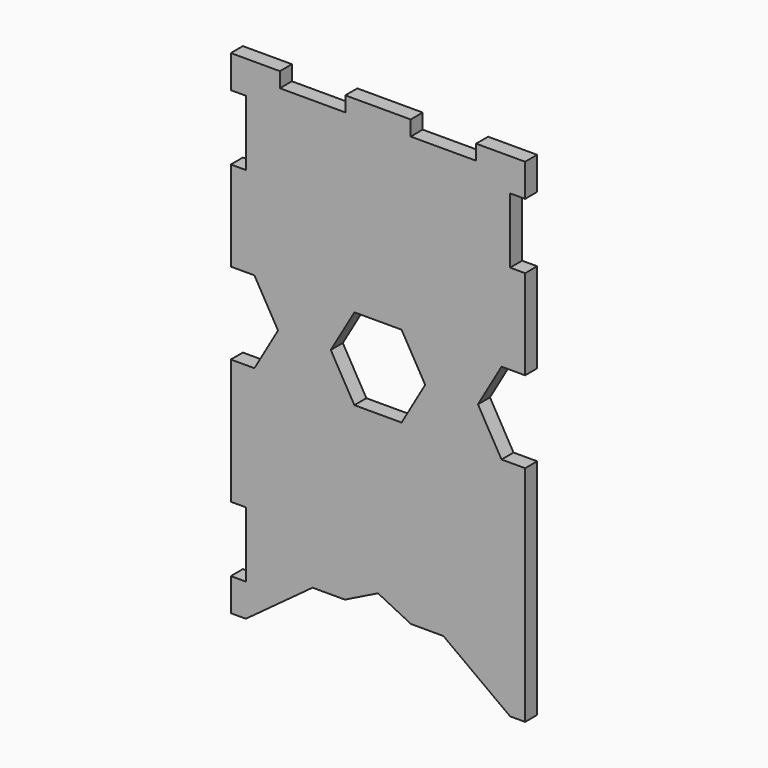
from build123d import *

# Parameters (mm, degrees)
F0_W     = 114.3
F0_H     = 191.516
F1_DEPTH = 5.842
F2_W     = 5.842
F2_H     = 25.4
F2_W_2   = 25.4
F2_H_2   = 5.842
F3_DEPTH = 5.842
F5_DEPTH = 5.842


# Not quite as in the source:
# - a feature names something its author has since deleted; it is built from what else it names


with BuildPart() as f1:
    # F0 (on Front) → F1 (new body)
    with BuildSketch(Plane.XZ):
        with Locations((-13.1958257407, -66.1412229082)):
            Rectangle(F0_W, F0_H)
    extrude(amount=-F1_DEPTH)

    # F2 (on face) → F3 (cut, through all)
    with BuildSketch(Plane.XZ):
        with Locations((-67.4248257407, 4.2167770918)):
            Rectangle(F2_W, F2_H)
        with Locations((-67.4248257407, -136.4992229082)):
            Rectangle(F2_W, F2_H)
        with Locations((41.0331742593, 4.2167770918)):
            Rectangle(F2_W, F2_H)
        with Locations((-38.5958257407, 26.6957770918)):
            Rectangle(F2_W_2, F2_H_2)
        with Locations((12.2041742593, 26.6957770918)):
            Rectangle(F2_W_2, F2_H_2)
        Polygon((-70.3458257407, -75.1582229082), (-70.3458257407, -43.4082229082), (-79.5112612641, -43.4082229082), (-88.6766967875, -59.2832229082), (-79.5112612641, -75.1582229082), align=None)
        Polygon((-61.1803902173, -43.4082229082), (-70.3458257407, -43.4082229082), (-70.3458257407, -75.1582229082), (-61.1803902173, -75.1582229082), (-52.0149546939, -59.2832229082), align=None)
        Polygon((43.9541742593, -75.1582229082), (43.9541742593, -43.4082229082), (34.7887387359, -43.4082229082), (25.6233032125, -59.2832229082), (34.7887387359, -75.1582229082), align=None)
        Polygon((53.1196097827, -43.4082229082), (43.9541742593, -43.4082229082), (43.9541742593, -75.1582229082), (53.1196097827, -75.1582229082), (62.2850453061, -59.2832229082), align=None)
        Polygon((-26.0228257407, -142.8492229082), (-64.5038257407, -161.8992229082), (38.1121742593, -161.8992229082), (-0.3688257407, -142.8492229082), align=None)
        Polygon((-13.1958257407, -136.4992229082), (-26.0228257407, -142.8492229082), (-0.3688257407, -142.8492229082), align=None)
        Polygon((-38.5958257407, -142.8492229082), (-64.5038257407, -161.8992229082), (-26.0228257407, -142.8492229082), align=None)
        Polygon((-0.3688257407, -142.8492229082), (38.1121742593, -161.8992229082), (12.2041742593, -142.8492229082), align=None)
    extrude(amount=-F3_DEPTH, mode=Mode.SUBTRACT)

    # F4 (on face) → F5 (cut, through all)
    with BuildSketch(Plane.XZ):
        Polygon((5.1350453061, -59.2832229082), (-4.0303902173, -43.4082229082), (-22.3612612641, -43.4082229082), (-31.5266967875, -59.2832229082), (-22.3612612641, -75.1582229082), (-4.0303902173, -75.1582229082), align=None)
    extrude(amount=-F5_DEPTH, mode=Mode.SUBTRACT)


solid = f1.part
